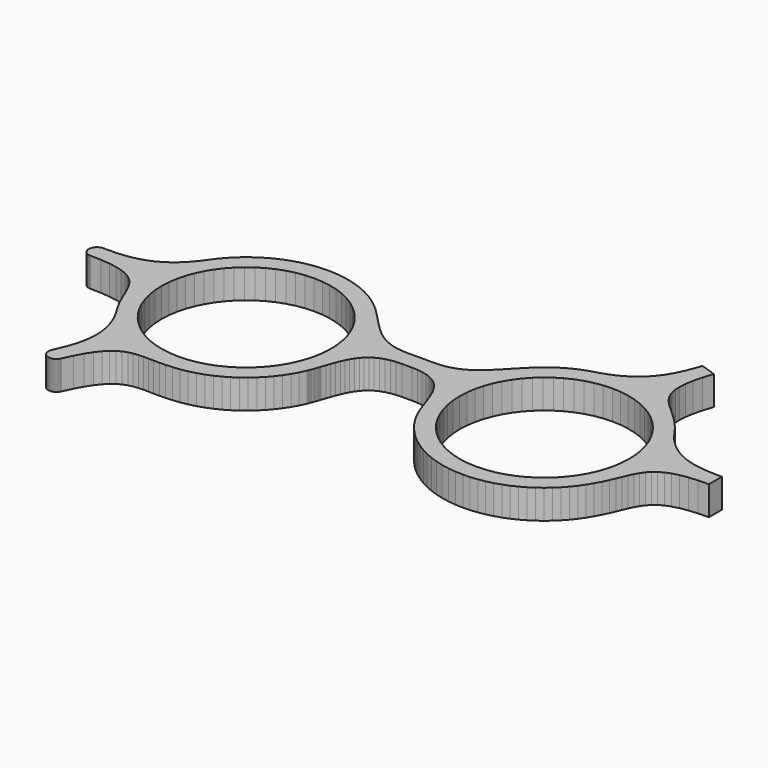
from build123d import *

# Parameters (mm, degrees)
F1_DEPTH = 6


with BuildPart() as f1:
    # F0 (on Top) → F1 (new body)
    with BuildSketch(Plane.XY):
        Polygon((48.825615, 11.044459), (48.832506, 11.034124), (48.83285, 11.034468), (48.832161, 11.035846), (48.830783, 11.038258), (48.828716, 11.041703), (48.82596, 11.045493), (48.823204, 11.049282), (48.820792, 11.053072), (48.818381, 11.056517), (48.816314, 11.059273), (48.81528, 11.060996), (48.814591, 11.06134), (48.81528, 11.060307), (48.817347, 11.057206), (48.820448, 11.052038), align=None)
    extrude(amount=F1_DEPTH)


with BuildPart() as f1b:
    # F0 (on Top) → F1, piece 2 (new body)
    with BuildSketch(Plane.XY):
        Polygon((-46.415772, 12.033546), (-47.157501, 11.034124), (-47.96951, 9.901032), (-48.796677, 8.885762), (-49.63797, 7.982114), (-50.49287, 7.18423), (-51.36069, 6.48522), (-52.240395, 5.878883), (-53.131641, 5.359362), (-54.033567, 4.919424), (-54.945312, 4.553555), (-55.866358, 4.254865), (-56.795845, 4.017498), (-57.733083, 3.834908), (-58.677211, 3.700894), (-59.627713, 3.608909), (-60.583727, 3.553099), (-61.544564, 3.526572), (-61.631725, 3.526227), (-61.719058, 3.525538), (-61.806391, 3.524849), (-61.893552, 3.52416), (-61.980713, 3.523471), (-62.068046, 3.523127), (-62.15538, 3.522782), (-62.242541, 3.522093), (-62.329701, 3.521404), (-62.417035, 3.52106), (-62.504368, 3.520715), (-62.591529, 3.520026), (-62.67869, 3.519337), (-62.766023, 3.518992), (-62.853356, 3.518648), (-62.940517, 3.517959), (-62.940517, 3.517614), (-62.940517, 3.51727), (-62.940517, 3.516925), (-63.111738, 3.508313), (-63.278136, 3.482819), (-63.438678, 3.441822), (-63.592501, 3.385323), (-63.738918, 3.314698), (-63.877066, 3.230983), (-64.005913, 3.13452), (-64.124941, 3.026344), (-64.233117, 2.907488), (-64.329579, 2.778297), (-64.413467, 2.640149), (-64.48392, 2.494077), (-64.540247, 2.340081), (-64.581416, 2.179539), (-64.60691, 2.013141), (-64.615522, 1.84192), (-64.60691, 1.670699), (-64.581416, 1.504301), (-64.540247, 1.343759), (-64.48392, 1.189763), (-64.413467, 1.043691), (-64.329579, 0.905543), (-64.233117, 0.776352), (-64.124941, 0.657496), (-64.005913, 0.54932), (-63.877066, 0.452858), (-63.738918, 0.369142), (-63.592501, 0.298517), (-63.438678, 0.242018), (-63.278136, 0.201021), (-63.111738, 0.175527), (-62.940517, 0.166915), (-62.940517, 0.16657), (-62.940517, 0.166226), (-62.940517, 0.165881), (-60.757877, 0.112138), (-58.879094, -0.047026), (-57.275402, -0.307131), (-55.917518, -0.664387), (-54.776846, -1.11535), (-53.82445, -1.655541), (-53.031389, -2.280826), (-52.368897, -2.988104), (-51.808035, -3.772897), (-51.320038, -4.63107), (-50.875793, -5.559179), (-50.446534, -6.552744), (-50.003494, -7.608321), (-49.517736, -8.721776), (-48.960147, -9.888975), (-48.301962, -11.106471), (-48.265788, -11.171584), (-48.22927, -11.236351), (-48.19258, -11.300775), (-48.155717, -11.365543), (-48.11851, -11.429621), (-48.081131, -11.494045), (-48.043407, -11.557779), (-48.005511, -11.621858), (-47.967443, -11.685247), (-47.92903, -11.748982), (-47.890445, -11.812371), (-47.851688, -11.875761), (-47.812758, -11.938806), (-47.773656, -12.001852), (-47.734382, -12.064897), (-47.694936, -12.127598), (-47.010395, -13.308576), (-46.436442, -14.456482), (-45.96722, -15.573727), (-45.597045, -16.662032), (-45.319887, -17.723122), (-45.130062, -18.758373), (-45.021197, -19.770197), (-44.987952, -20.760662), (-45.024126, -21.731146), (-45.123861, -22.683026), (-45.281474, -23.618369), (-45.490936, -24.539588), (-45.74639, -25.447715), (-46.042151, -26.344818), (-46.372019, -27.233308), (-46.730309, -28.114219), (-46.764932, -28.194145), (-46.799556, -28.274416), (-46.834007, -28.354686), (-46.86863, -28.434613), (-46.903253, -28.514539), (-46.937704, -28.59481), (-46.972327, -28.67508), (-47.00695, -28.755007), (-47.041574, -28.834933), (-47.076197, -28.915203), (-47.110648, -28.995474), (-47.145271, -29.0754), (-47.179894, -29.155671), (-47.214345, -29.235942), (-47.248968, -29.315868), (-47.283591, -29.396139), (-47.283591, -29.396483), (-47.283419, -29.396483), (-47.283247, -29.396483), (-47.283075, -29.396483), (-47.282902, -29.396483), (-47.343881, -29.55668), (-47.387461, -29.719289), (-47.414161, -29.882586), (-47.424496, -30.046228), (-47.418639, -30.208837), (-47.397452, -30.368689), (-47.360934, -30.525786), (-47.309774, -30.678059), (-47.244317, -30.82482), (-47.16508, -30.965035), (-47.072235, -31.097671), (-46.96647, -31.221006), (-46.848304, -31.334694), (-46.717907, -31.436669), (-46.575797, -31.52693), (-46.422318, -31.603756), (-46.262121, -31.664734), (-46.099512, -31.708142), (-45.936042, -31.735014), (-45.772573, -31.745005), (-45.610136, -31.739493), (-45.449939, -31.718133), (-45.293015, -31.681271), (-45.140742, -31.630283), (-44.993981, -31.564826), (-44.853766, -31.485589), (-44.721474, -31.392916), (-44.597967, -31.287152), (-44.484624, -31.168985), (-44.382304, -31.038416), (-44.292215, -30.896478), (-44.215389, -30.743171), (-44.215389, -30.743516), (-44.215217, -30.743516), (-44.215045, -30.743516), (-44.214873, -30.743516), (-44.2147, -30.743516), (-44.2147, -30.74386), (-43.302095, -28.795314), (-42.41481, -27.15786), (-41.544924, -25.804627), (-40.6852, -24.708742), (-39.827544, -23.843678), (-38.964547, -23.18222), (-38.088804, -22.698529), (-37.192218, -22.365043), (-36.267554, -22.155237), (-35.306889, -22.042582), (-34.302816, -22.000552), (-33.247411, -22.00193), (-32.133267, -22.020189), (-30.952633, -22.028458), (-29.698102, -21.999863), (-28.361577, -21.908568), (-26.889487, -21.748371), (-25.449438, -21.487922), (-24.045044, -21.131355), (-22.679753, -20.68177), (-21.357181, -20.142957), (-20.081118, -19.518706), (-18.854836, -18.812461), (-17.682298, -18.028013), (-16.566776, -17.168461), (-15.51206, -16.237941), (-14.521595, -15.239552), (-13.59917, -14.177429), (-12.748232, -13.055017), (-11.972396, -11.876106), (-11.275453, -10.643795), (-10.660504, -9.361875), (-10.653097, -9.343272), (-10.63191, -9.290217), (-10.598664, -9.206157), (-10.554567, -9.094191), (-10.501513, -8.958454), (-10.440879, -8.802392), (-10.374389, -8.629448), (-10.303248, -8.443068), (-10.22935, -8.247042), (-10.154075, -8.04516), (-10.079144, -7.840521), (-10.005936, -7.636916), (-9.936173, -7.438134), (-9.871233, -7.247275), (-9.812838, -7.06813), (-9.762368, -6.904144), (-9.454893, -6.006008), (-9.149657, -5.12992), (-8.837704, -4.280359), (-8.510592, -3.462838), (-8.15902, -2.682179), (-7.774375, -1.943206), (-7.3477, -1.251087), (-6.87021, -0.610988), (-6.333292, -0.027389), (-5.727816, 0.494543), (-5.044998, 0.949985), (-4.276053, 1.333768), (-3.412195, 1.640726), (-2.44464, 1.866036), (-1.364431, 2.004873), (-0.162609, 2.052415), (-0.037552, 2.052415), (0.087505, 2.052415), (0.212562, 2.052415), (0.337619, 2.052415), (0.462676, 2.052415), (0.587733, 2.052415), (0.712445, 2.052415), (0.837502, 2.052415), (0.962559, 2.052415), (1.087272, 2.052415), (1.212329, 2.052415), (1.337386, 2.052415), (1.462443, 2.052415), (1.5875, 2.052415), (1.712557, 2.052415), (1.837613, 2.052415), (3.039607, 2.004873), (4.119645, 1.866036), (5.087028, 1.640726), (5.951057, 1.333768), (6.720003, 0.949985), (7.402821, 0.494543), (8.008469, -0.027389), (8.545214, -0.610988), (9.022705, -1.251087), (9.449552, -1.943206), (9.834369, -2.682179), (10.185769, -3.462838), (10.513053, -4.280359), (10.824834, -5.12992), (11.13007, -6.006008), (11.437372, -6.904144), (11.493527, -7.057795), (11.549338, -7.211446), (11.605493, -7.365098), (11.661648, -7.518749), (11.717803, -7.6724), (11.773958, -7.826051), (11.830113, -7.979703), (11.886268, -8.133009), (11.942423, -8.286316), (11.998578, -8.439967), (12.054733, -8.593619), (12.110888, -8.74727), (12.167043, -8.900921), (12.223198, -9.054573), (12.279353, -9.208224), (12.335508, -9.361875), (12.992833, -10.724755), (13.743174, -12.03148), (14.582055, -13.277571), (15.505685, -14.458205), (16.509242, -15.569593), (17.588246, -16.607255), (18.738563, -17.56637), (19.95606, -18.443491), (21.236257, -19.233796), (22.574677, -19.932461), (23.967184, -20.535698), (25.409301, -21.039026), (26.896549, -21.437968), (28.424793, -21.72839), (29.9899, -21.905812), (31.587391, -21.966101), (33.057069, -21.915114), (34.500219, -21.765252), (35.912708, -21.518928), (37.29178, -21.180275), (38.6333, -20.75205), (39.934513, -20.238386), (41.191628, -19.641695), (42.401546, -18.966112), (43.56082, -18.214392), (44.666352, -17.39067), (45.71435, -16.497357), (46.701369, -15.538931), (47.624311, -14.517805), (48.480417, -13.437423), (49.265554, -12.30192), (49.975933, -11.114051), (50.633946, -9.896554), (51.191707, -8.728666), (51.677465, -7.614867), (52.120849, -6.558945), (52.550108, -5.564691), (52.994525, -4.636238), (53.482695, -3.777375), (54.043557, -2.991893), (54.706049, -2.284271), (55.49911, -1.657952), (56.451679, -1.117073), (57.59235, -0.665765), (58.950406, -0.30782), (60.554098, -0.04737), (62.433053, 0.111793), (64.615521, 0.165881), (64.615521, 0.538985), (64.615521, 0.848699), (64.615521, 1.103292), (64.615521, 1.312409), (64.615521, 1.484664), (64.615521, 1.629358), (64.615521, 1.755448), (64.615521, 1.871203), (64.615521, 1.98627), (64.615521, 2.109259), (64.615521, 2.24913), (64.615521, 2.415184), (64.615521, 2.616033), (64.615521, 2.860979), (64.615521, 3.158636), (64.615521, 3.517959), (63.553743, 3.526227), (62.498166, 3.5562), (61.450168, 3.616833), (60.410782, 3.716052), (59.379665, 3.862813), (58.358539, 4.065729), (57.347404, 4.332724), (56.347292, 4.672755), (55.359239, 5.09409), (54.383243, 5.605342), (53.421028, 6.21478), (52.472249, 6.931015), (51.538628, 7.762661), (50.620166, 8.717986), (49.717895, 9.805603), (48.832506, 11.034124), (48.73432, 11.173995), (48.634757, 11.312832), (48.534505, 11.450636), (48.432874, 11.587751), (48.330211, 11.723832), (48.226513, 11.859224), (48.121438, 11.993583), (48.015329, 12.127253), (47.908186, 12.260233), (47.800355, 12.391836), (47.691145, 12.52275), (47.581247, 12.652974), (47.46997, 12.782165), (47.35766, 12.910667), (47.244661, 13.038136), (47.130628, 13.164571), (47.132351, 13.164226), (47.133729, 13.163537), (47.135107, 13.163193), (47.136485, 13.162848), (47.137863, 13.162504), (47.139241, 13.162159), (47.140619, 13.161815), (47.141997, 13.16147), (47.143375, 13.161126), (47.144753, 13.160781), (47.146131, 13.160092), (47.147509, 13.159748), (47.148887, 13.159403), (47.150265, 13.158714), (47.151643, 13.15837), (47.153366, 13.158025), (46.214577, 14.174673), (45.289914, 15.080388), (44.3935, 15.900666), (43.537394, 16.661687), (42.735376, 17.389636), (42.000537, 18.11035), (41.345969, 18.850356), (40.784418, 19.635149), (40.329321, 20.491255), (39.993424, 21.444169), (39.790163, 22.520417), (39.732286, 23.745837), (39.832883, 25.146613), (40.10539, 26.748238), (40.562898, 28.577584), (41.218155, 30.660144), (40.865033, 30.780894), (40.5722, 30.880974), (40.331043, 30.963484), (40.133295, 31.031181), (39.970342, 31.086991), (39.833572, 31.133844), (39.714371, 31.174496), (39.604817, 31.212048), (39.495952, 31.249255), (39.379508, 31.289046), (39.247216, 31.334349), (39.09012, 31.388092), (38.899951, 31.453205), (38.66844, 31.53227), (38.386976, 31.62856), (38.046601, 31.745004), (37.704503, 30.769009), (37.345179, 29.80576), (36.961051, 28.858187), (36.544883, 27.929733), (36.090131, 27.023329), (35.588525, 26.142246), (35.033865, 25.289584), (34.418226, 24.468618), (33.734719, 23.682792), (32.976454, 22.934517), (32.136195, 22.227584), (31.206363, 21.565092), (30.179725, 20.950142), (29.049389, 20.385491), (27.808121, 19.875272), (26.448687, 19.421898), (25.744509, 19.231039), (25.050667, 19.016755), (24.36716, 18.779043), (23.693988, 18.518938), (23.03253, 18.236785), (22.382785, 17.932583), (21.745098, 17.607366), (21.120502, 17.261134), (20.508997, 16.894576), (19.910929, 16.508381), (19.326985, 16.102548), (18.757511, 15.677768), (18.203195, 15.234384), (17.664382, 14.772741), (17.141417, 14.293529), (16.634988, 13.797435), (15.849506, 13.014709), (15.099164, 12.241285), (14.375349, 11.48302), (13.669794, 10.745425), (12.974229, 10.034702), (12.280387, 9.356018), (11.579654, 8.714886), (10.863764, 8.117161), (10.124446, 7.568702), (9.353434, 7.07502), (8.542458, 6.641972), (7.682907, 6.274724), (6.766167, 5.979135), (5.784659, 5.761405), (4.729427, 5.626357), (3.592201, 5.580193), (3.248036, 5.580193), (2.903526, 5.580193), (2.559016, 5.580193), (2.214851, 5.580193), (1.870686, 5.580193), (1.526177, 5.580193), (1.181667, 5.580193), (0.837502, 5.580193), (0.493337, 5.580193), (0.148828, 5.580193), (-0.19551, 5.580193), (-0.539847, 5.580193), (-0.884184, 5.580193), (-1.228521, 5.580193), (-1.572859, 5.580193), (-1.917196, 5.580193), (-3.054422, 5.626357), (-4.109655, 5.761405), (-5.091335, 5.979135), (-6.007902, 6.274724), (-6.867454, 6.641972), (-7.678602, 7.07502), (-8.449614, 7.568702), (-9.188931, 8.117161), (-9.904822, 8.714886), (-10.605382, 9.356018), (-11.299225, 10.034702), (-11.994789, 10.745425), (-12.700345, 11.48302), (-13.42416, 12.241285), (-14.174501, 13.014709), (-14.959983, 13.797435), (-15.692066, 14.504713), (-16.457394, 15.175818), (-17.254933, 15.81006), (-18.082962, 16.406061), (-18.940446, 16.9621), (-19.825836, 17.477141), (-20.73758, 17.949464), (-21.674646, 18.378034), (-22.635484, 18.761128), (-23.618714, 19.098059), (-24.622959, 19.386758), (-25.647014, 19.625847), (-26.689155, 19.814294), (-27.748522, 19.950375), (-28.823392, 20.033402), (-29.912387, 20.061307), (-31.239954, 20.019966), (-32.545645, 19.896976), (-33.827221, 19.695438), (-35.082097, 19.417419), (-36.30769, 19.06533), (-37.50176, 18.642273), (-38.661723, 18.149969), (-39.784997, 17.591863), (-40.86934, 16.969679), (-41.911999, 16.285827), (-42.910732, 15.543065), (-43.862956, 14.744147), (-44.766088, 13.891141), (-45.617888, 12.986804), align=None)
        Polygon((-12.42646, -0.952397), (-12.516894, -2.737645), (-12.782338, -4.472251), (-13.213836, -6.146567), (-13.802776, -7.752326), (-14.540026, -9.280571), (-15.416803, -10.722343), (-16.424321, -12.068687), (-17.553795, -13.310988), (-18.796097, -14.44029), (-20.142612, -15.447981), (-21.584385, -16.324758), (-23.112629, -17.062008), (-24.718216, -17.650775), (-26.392705, -18.082445), (-28.126966, -18.347718), (-29.912387, -18.438324), (-31.697807, -18.347718), (-33.432068, -18.082445), (-35.106557, -17.650775), (-36.712144, -17.062008), (-38.240388, -16.324758), (-39.682161, -15.447981), (-41.028676, -14.44029), (-42.270978, -13.310988), (-43.400452, -12.068687), (-44.40797, -10.722343), (-45.284747, -9.280571), (-46.021998, -7.752326), (-46.610937, -6.146567), (-47.042435, -4.472251), (-47.307879, -2.737645), (-47.398313, -0.952397), (-47.307879, 0.832852), (-47.042435, 2.567113), (-46.610937, 4.241429), (-46.021998, 5.847188), (-45.284747, 7.375432), (-44.40797, 8.817205), (-43.400452, 10.163548), (-42.270978, 11.40585), (-41.028676, 12.535152), (-39.682161, 13.542842), (-38.240388, 14.419619), (-36.712144, 15.15687), (-35.106557, 15.745636), (-33.432068, 16.177307), (-31.697807, 16.442579), (-29.912387, 16.533185), (-28.126966, 16.442579), (-26.392705, 16.177307), (-24.718216, 15.745636), (-23.112629, 15.15687), (-21.584385, 14.419619), (-20.142612, 13.542842), (-18.796097, 12.535152), (-17.553795, 11.40585), (-16.424321, 10.163548), (-15.416803, 8.817205), (-14.540026, 7.375432), (-13.802776, 5.847188), (-13.213836, 4.241429), (-12.782338, 2.567113), (-12.516894, 0.832852), align=None, mode=Mode.SUBTRACT)
        Polygon((49.073318, -0.952397), (48.982712, -2.737645), (48.717439, -4.472251), (48.285769, -6.146567), (47.697002, -7.752326), (46.959752, -9.280571), (46.082975, -10.722343), (45.075284, -12.068687), (43.945982, -13.310988), (42.703681, -14.44029), (41.357337, -15.447981), (39.915565, -16.324758), (38.387321, -17.062008), (36.781562, -17.650775), (35.107245, -18.082445), (33.37264, -18.347718), (31.587391, -18.438324), (29.802143, -18.347718), (28.067537, -18.082445), (26.393221, -17.650775), (24.787462, -17.062008), (23.259217, -16.324758), (21.817445, -15.447981), (20.471101, -14.44029), (19.2288, -13.310988), (18.099498, -12.068687), (17.091807, -10.722343), (16.21503, -9.280571), (15.47778, -7.752326), (14.889013, -6.146567), (14.457343, -4.472251), (14.19207, -2.737645), (14.101464, -0.952397), (14.19207, 0.832852), (14.457343, 2.567113), (14.889013, 4.241429), (15.47778, 5.847188), (16.21503, 7.375432), (17.091807, 8.817205), (18.099498, 10.163548), (19.2288, 11.40585), (20.471101, 12.535152), (21.817445, 13.542842), (23.259217, 14.419619), (24.787462, 15.15687), (26.393221, 15.745636), (28.067537, 16.177307), (29.802143, 16.442579), (31.587391, 16.533185), (33.37264, 16.442579), (35.107245, 16.177307), (36.781562, 15.745636), (38.387321, 15.15687), (39.915565, 14.419619), (41.357337, 13.542842), (42.703681, 12.535152), (43.945982, 11.40585), (45.075284, 10.163548), (46.082975, 8.817205), (46.959752, 7.375432), (47.697002, 5.847188), (48.285769, 4.241429), (48.717439, 2.567113), (48.982712, 0.832852), align=None, mode=Mode.SUBTRACT)
    extrude(amount=F1_DEPTH)


solid = Compound([f1.part, f1b.part])
